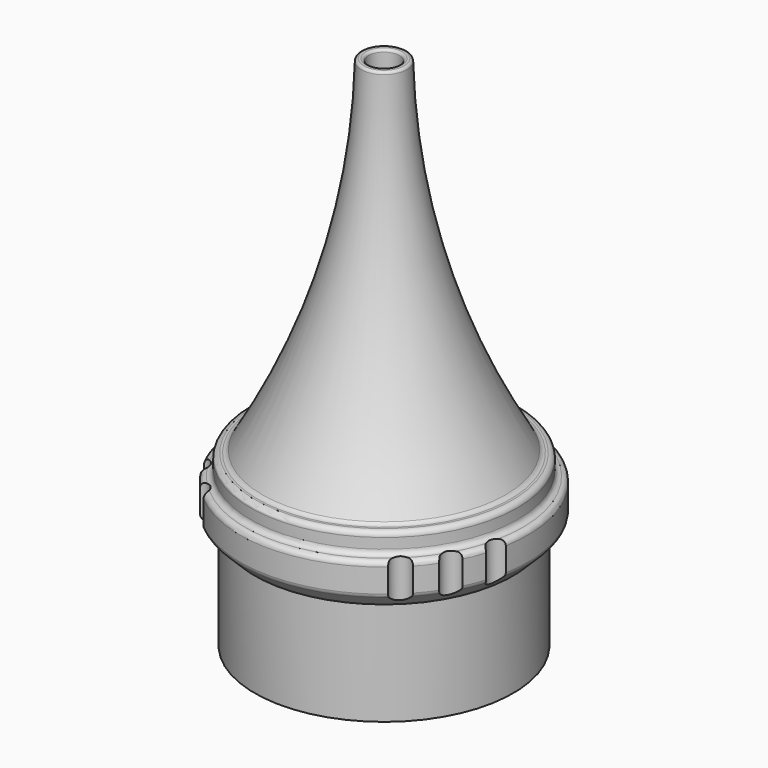
from build123d import *

# Parameters (mm, degrees)
F3_R     = 0.49999
F4_R     = 0.25
F5_R     = 1
F6_DEPTH = 25


# Not quite as in the source:
# - a fillet or chamfer is up to 0.001 mm smaller than in the source, because OpenCascade refuses the exact size


with BuildPart() as f2:
    # F0 (on Front) → F2 (revolve)
    with BuildSketch(Plane.XZ):
        with BuildLine():
            ThreePointArc((-2.2, 50), (-4.8442723557, 32.5670757303), (-11.9142135624, 16.4142135624))
            Line((-11.9142135624, 16.4142135624), (-12.9142135624, 16.4142135624))
            Line((-12.9142135624, 16.4142135624), (-12.9142135624, 14.4142135624))
            Line((-12.9142135624, 14.4142135624), (-13.9142135624, 14.4142135624))
            Line((-13.9142135624, 14.4142135624), (-13.9142135624, 11.4142135624))
            Line((-13.9142135624, 11.4142135624), (-12.5, 10))
            Line((-12.5, 10), (-12.5, 0))
            Line((-12.5, 0), (-10.5, 0))
            Line((-10.5, 0), (-10.5, 9))
            ThreePointArc((-10.5, 9), (-10.1394101324, 12.5845638892), (-9.0909232783, 16.0312722674))
            ThreePointArc((-9.0909232783, 16.0312722674), (-9.0063513538, 16.2244885639), (-8.9142135624, 16.4142135624))
            ThreePointArc((-8.9142135624, 16.4142135624), (-3.0579407905, 32.732668713), (-1.5, 50))
            Line((-1.5, 50), (-2.2, 50))
        make_face()
    revolve(axis=Axis((0, 0, 0), (0, 0, 1)))

    # F3 (radius 0.5 in the source; OpenCascade refuses exactly that, so slightly less here)
    f3_edges = [f2.edges().sort_by_distance(p)[0] for p in [
        (13.914214, 0, 14.414214),
        (13.914214, 0, 11.414214),
        (12.914214, 0, 16.414214),
        (11.914214, 0, 16.414214),
        (12.914214, 0, 14.414214),
    ]]
    fillet(f3_edges, radius=F3_R)

    # F4
    f4_edges = [f2.edges().sort_by_distance(p)[0] for p in [
        (2.2, 0, 50),
        (1.5, 0, 50),
    ]]
    fillet(f4_edges, radius=F4_R)

    # F5 (on Top) → F6 (cut)
    with BuildSketch(Plane.XY):
        with Locations((0, 14.2142135624)):
            Circle(F5_R)
        with Locations((-3.9602067, 13.6513966352)):
            Circle(F5_R)
        with Locations((3.9602067, 13.6513966352)):
            Circle(F5_R)
        with Locations((-9.8423529332, -10.255337924)):
            Circle(F5_R)
        with Locations((-12.3098700398, -7.1071067812)):
            Circle(F5_R)
        with Locations((-13.8025596332, -3.3960587112)):
            Circle(F5_R)
        with Locations((13.8025596332, -3.3960587112)):
            Circle(F5_R)
        with Locations((12.3098700398, -7.1071067812)):
            Circle(F5_R)
        with Locations((9.8423529332, -10.255337924)):
            Circle(F5_R)
    extrude(amount=F6_DEPTH, mode=Mode.SUBTRACT)


solid = f2.part
